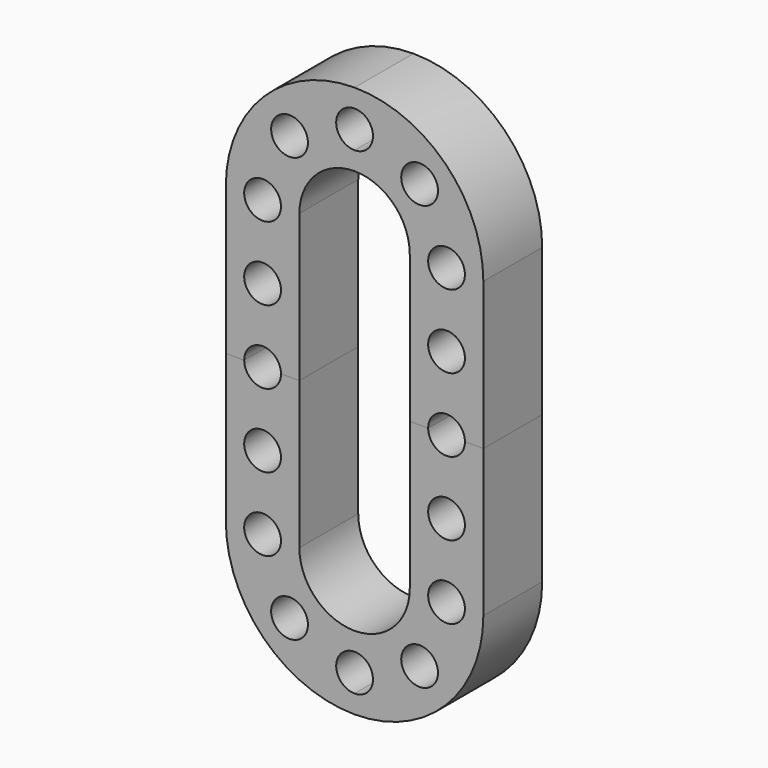
from build123d import *
from build123d import SkipClean  # not in build123d's __all__

# Parameters (mm, degrees)
F0_R     = 5
F1_DEPTH = 20


with BuildPart() as f1:
    # F0 (on Front) → F1 (new body)
    with BuildSketch(Plane.XZ):
        with BuildLine():
            ThreePointArc((-15, 40), (-10.6066017178, 50.6066017178), (0, 55))
            Line((0, 55), (0.0401919294, 60.0001615417))
            ThreePointArc((0.0401919294, 60.0001615417), (-4.9999596144, 64.979903873), (0, 70))
            Line((0, 70), (0, 75))
            ThreePointArc((0, 75), (-24.7487373415, 64.7487373415), (-35, 40))
            Line((-35, 40), (-35, 0))
            Line((-35, 0), (-30, 0))
            ThreePointArc((-30, 0), (-25, 5), (-20, 0))
            Line((-20, 0), (-15, 0))
            Line((-15, 0), (-15, 40))
        make_face()
        with Locations((-25, 20)):
            Circle(F0_R, mode=Mode.SUBTRACT)
        with Locations((-25, 40)):
            Circle(F0_R, mode=Mode.SUBTRACT)
        with Locations((-17.6776695297, 57.6776695297)):
            Circle(F0_R, mode=Mode.SUBTRACT)
    extrude(amount=F1_DEPTH)

    # F2: F1 across plane


with BuildPart() as f1_1:
    add(f1.part, clean=False)
    add(f1.part.mirror(Plane.YZ), clean=False)

    # F3: F1 across plane


with BuildPart() as f1_2:
    add(f1_1.part, clean=False)
    with SkipClean():  # cleaning this boolean's faces spoils the solid; the shape is the same uncleaned
        add(f1_1.part.mirror(Plane.XY), clean=False)


solid = f1_2.part
